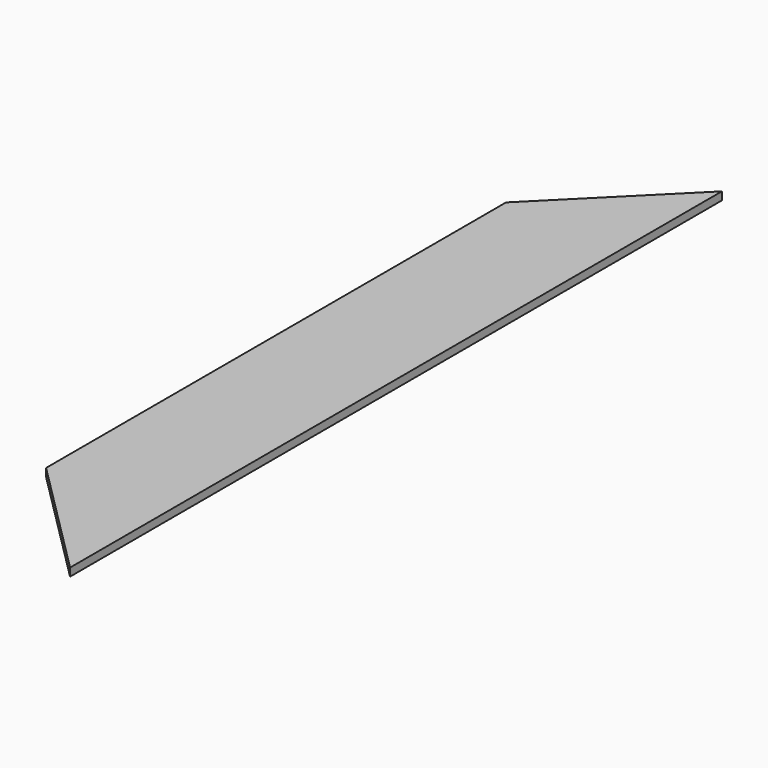
from build123d import *

# Parameters (mm, degrees)
F0_W          = 150
F0_H          = 10
F1_DEPTH      = 1019
F3_DEPTH      = 10.001
F3_DEPTH_BACK = 1540
F5_DEPTH      = 1577
F5_DEPTH_BACK = 10.001


# Not quite as in the source:
# - an extrude ends at something that could not be found from the text; its depth is read off the source's solid


with BuildPart() as f1:
    # F0 (on Front) → F1 (new body)
    with BuildSketch(Plane.XZ):
        with Locations((0.4800241441, -31.7408985884)):
            Rectangle(F0_W, F0_H)
    extrude(amount=F1_DEPTH)

    # F2 (on face) → F3 (cut, two sides)
    with BuildSketch(Plane.XY.offset(-26.7408985884)) as f3_sk:
        Polygon((-74.5199758559, -150), (75.4800241441, 0), (178.0070960522, 169.0949052572), (-164.1357541084, 159.836769104), (-164.1357541084, -150), (-107.9861149192, -156.7480415106), align=None)
    extrude(amount=-F3_DEPTH, mode=Mode.SUBTRACT)
    extrude(f3_sk.sketch, amount=F3_DEPTH_BACK, mode=Mode.SUBTRACT)

    # F4 (on face) → F5 (cut, two sides)
    with BuildSketch(Plane.XY.offset(-26.7408985884)) as f5_sk:
        Polygon((72.7586299181, -1200.1620531082), (75.4800241441, -1019), (-74.5199758559, -869), (-237.236186862, -869), (-237.236186862, -1200.1620531082), align=None)
    extrude(amount=F5_DEPTH, mode=Mode.SUBTRACT)
    extrude(f5_sk.sketch, amount=-F5_DEPTH_BACK, mode=Mode.SUBTRACT)


solid = f1.part
